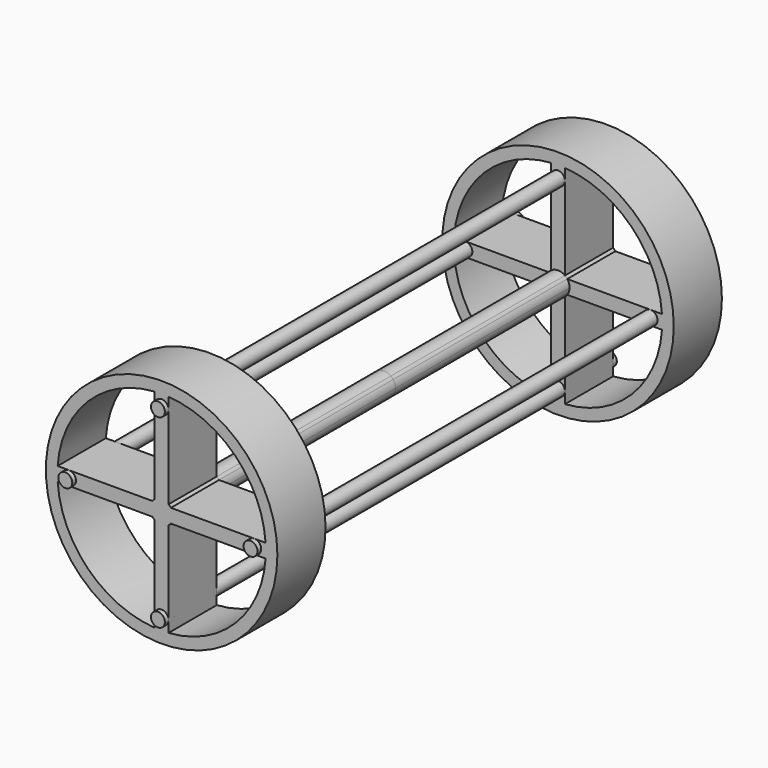
from build123d import *
from build123d import SkipClean  # not in build123d's __all__

# Parameters (mm, degrees)
F0_R          = 250
F1_DEPTH      = 600
F1_DEPTH_BACK = 600
F3_DEPTH      = 600.001
F3_DEPTH_BACK = 600.001
F4_R          = 250
F4_R_2        = 25
F5_DEPTH      = 470
F5_DEPTH_BACK = 470
F6_R          = 15
F7_DEPTH      = 610
F7_DEPTH_BACK = 610


with BuildPart() as f1:
    # F0 (on Front) → F1 (new body, two sides)
    with BuildSketch(Plane.XZ) as f1_sk:
        Circle(F0_R)
    extrude(amount=F1_DEPTH)
    extrude(f1_sk.sketch, amount=-F1_DEPTH_BACK)

    # F2 (on Front) → F3 (cut, two sides)
    with BuildSketch(Plane.XZ) as f3_sk:
        with BuildLine():
            Line((20, 15), (224.4994432064, 15))
            ThreePointArc((224.4994432064, 15), (159.099025767, 159.099025767), (15, 224.4994432064))
            Line((15, 224.4994432064), (15, 20))
            ThreePointArc((15, 20), (17.6776695297, 17.6776695297), (20, 15))
        make_face()
        with BuildLine():
            Line((-15, 20), (-15, 224.4994432064))
            ThreePointArc((-15, 224.4994432064), (-159.099025767, 159.099025767), (-224.4994432064, 15))
            Line((-224.4994432064, 15), (-20, 15))
            ThreePointArc((-20, 15), (-17.6776695297, 17.6776695297), (-15, 20))
        make_face()
        with BuildLine():
            ThreePointArc((-224.4994432064, -15), (-159.099025767, -159.099025767), (-15, -224.4994432064))
            Line((-15, -224.4994432064), (-15, -20))
            ThreePointArc((-15, -20), (-17.6776695297, -17.6776695297), (-20, -15))
            Line((-20, -15), (-224.4994432064, -15))
        make_face()
        with BuildLine():
            ThreePointArc((15, -224.4994432064), (159.099025767, -159.099025767), (224.4994432064, -15))
            Line((224.4994432064, -15), (20, -15))
            ThreePointArc((20, -15), (17.6776695297, -17.6776695297), (15, -20))
            Line((15, -20), (15, -224.4994432064))
        make_face()
    extrude(amount=F3_DEPTH, mode=Mode.SUBTRACT)
    extrude(f3_sk.sketch, amount=-F3_DEPTH_BACK, mode=Mode.SUBTRACT)

    # F4 (on Front) → F5 (cut, two sides)
    with BuildSketch(Plane.XZ) as f5_sk:
        Circle(F4_R)
        Circle(F4_R_2, mode=Mode.SUBTRACT)
    with SkipClean():  # cleaning this boolean's faces spoils the solid; the shape is the same uncleaned
        extrude(amount=-F5_DEPTH, mode=Mode.SUBTRACT)
        extrude(f5_sk.sketch, amount=F5_DEPTH_BACK, mode=Mode.SUBTRACT)


with BuildPart() as f7:
    # F6 (on Front) → F7 (new body, two sides)
    with BuildSketch(Plane.XZ) as f7_sk:
        with Locations((0, 200)):
            Circle(F6_R)
    extrude(amount=F7_DEPTH)
    extrude(f7_sk.sketch, amount=-F7_DEPTH_BACK)


with BuildPart() as f7b:
    # F6 (on Front) → F7, piece 2 (new body, two sides)
    with BuildSketch(Plane.XZ) as f7_2_sk:
        with Locations((-200, 0)):
            Circle(F6_R)
    extrude(amount=F7_DEPTH)
    extrude(f7_2_sk.sketch, amount=-F7_DEPTH_BACK)


with BuildPart() as f7c:
    # F6 (on Front) → F7, piece 3 (new body, two sides)
    with BuildSketch(Plane.XZ) as f7_3_sk:
        with Locations((0, -200)):
            Circle(F6_R)
    extrude(amount=F7_DEPTH)
    extrude(f7_3_sk.sketch, amount=-F7_DEPTH_BACK)


with BuildPart() as f7d:
    # F6 (on Front) → F7, piece 4 (new body, two sides)
    with BuildSketch(Plane.XZ) as f7_4_sk:
        with Locations((200, 0)):
            Circle(F6_R)
    extrude(amount=F7_DEPTH)
    extrude(f7_4_sk.sketch, amount=-F7_DEPTH_BACK)


solid = Compound([f1.part, f7.part, f7b.part, f7c.part, f7d.part])
